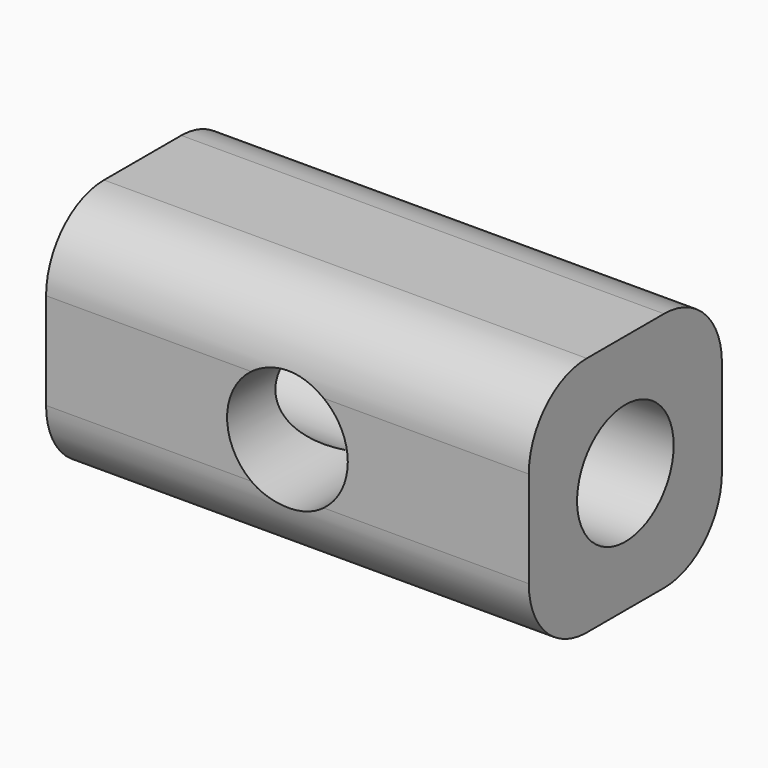
from build123d import *

# Parameters (mm, degrees)
F0_W          = 20
F0_H          = 10
F1_DEPTH      = 10
F2_R          = 2.5
F3_DEPTH      = 8
F4_R          = 2.5
F5_DEPTH      = 10.001
F5_DEPTH_BACK = 10.001
F6_T1_DEPTH   = 35


# Not quite as in the source:
# - a fillet or chamfer that OpenCascade refuses, or shapes differently, is made with other operations: its cross-section is extruded or revolved along the edge and cut away or added


with BuildPart() as f1:
    # F0 (on Front) → F1 (new body)
    with BuildSketch(Plane.XZ):
        with Locations((0, 5)):
            Rectangle(F0_W, F0_H)
    extrude(amount=F1_DEPTH)

    # F2 (on face) → F3 (cut)
    with BuildSketch(Plane.XZ.offset(10)):
        with Locations((0, 5)):
            Circle(F2_R)
    extrude(amount=-F3_DEPTH, mode=Mode.SUBTRACT)

    # F4 (on Right) → F5 (cut, two sides)
    with BuildSketch(Plane.YZ) as f5_sk:
        with Locations((-5, 5)):
            Circle(F4_R)
    extrude(amount=-F5_DEPTH, mode=Mode.SUBTRACT)
    extrude(f5_sk.sketch, amount=F5_DEPTH_BACK, mode=Mode.SUBTRACT)

    # F6: fillet of radius 3 on 4 edges, made by hand

    # F6_s2 → F6_t1 (cut)
    with BuildSketch(Plane.YZ.offset(-17.5)):
        with BuildLine():
            ThreePointArc((-3, 10), (-0.8786796564, 9.1213203436), (0, 7))
            Line((0, 7), (0, 10))
            Line((0, 10), (-3, 10))
        make_face()
        with BuildLine():
            ThreePointArc((-7, 10), (-9.1213203436, 9.1213203436), (-10, 7))
            Line((-10, 7), (-10, 10))
            Line((-10, 10), (-7, 10))
        make_face()
        with BuildLine():
            ThreePointArc((-10, 3), (-9.1213203436, 0.8786796564), (-7, 0))
            Line((-7, 0), (-10, 0))
            Line((-10, 0), (-10, 3))
        make_face()
        with BuildLine():
            ThreePointArc((0, 3), (-0.8786796564, 0.8786796564), (-3, 0))
            Line((-3, 0), (0, 0))
            Line((0, 0), (0, 3))
        make_face()
    extrude(amount=F6_T1_DEPTH, mode=Mode.SUBTRACT)


solid = f1.part
